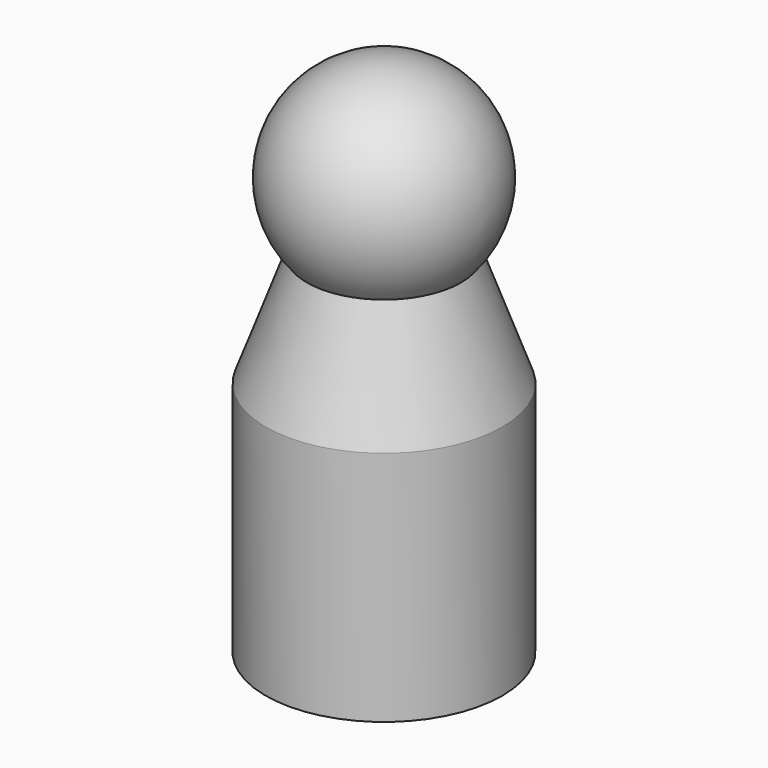
from build123d import *

# Parameters (mm, degrees)
F0_R      = 7.5
F1_DEPTH  = 15
F1_FACE_R = 7.5
F2_DEPTH  = 10
F2_TAPER  = 20


# Not quite as in the source:
# - a feature names something its author has since deleted; it is built from what else it names


with BuildPart() as f1:
    # F0 (on Top) → F1 (new body)
    with BuildSketch(Plane.XY):
        Circle(F0_R)
    extrude(amount=F1_DEPTH)

    # F1_face (on face) → F2 (join)
    with BuildSketch(Plane.XY.offset(15)):
        Circle(F1_FACE_R)
    extrude(amount=F2_DEPTH, taper=F2_TAPER)

    # F3 (on Front) → F4 (revolve)
    with BuildSketch(Plane.XZ):
        with BuildLine():
            Line((0, 33), (0, 20))
            ThreePointArc((0, 20), (6.5, 26.5), (0, 33))
        make_face()
    revolve(axis=Axis((0, 0, 26.5), (0, 0, 1)))


solid = f1.part
